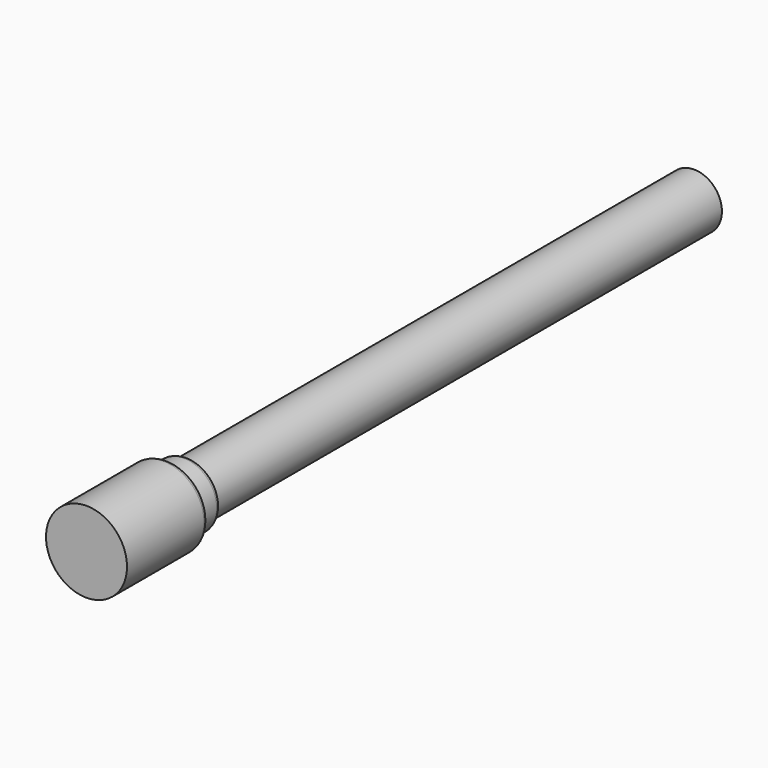
from build123d import *

# Parameters (mm, degrees)
F0_R     = 11
F1_DEPTH = 250
F2_R     = 13
F2_R_2   = 11
F3_DEPTH = 10
F4_R     = 1.99999
F5_R     = 16
F5_R_2   = 13
F6_DEPTH = 40
F7_R     = 2


# Not quite as in the source:
# - a fillet or chamfer is up to 0.001 mm smaller than in the source, because OpenCascade refuses the exact size


with BuildPart() as f1:
    # F0 (on Front) → F1 (new body)
    with BuildSketch(Plane.XZ):
        Circle(F0_R)
    extrude(amount=F1_DEPTH)

    # F2 (on face) → F3 (join)
    with BuildSketch(Plane.XZ.offset(250)):
        Circle(F2_R)
        Circle(F2_R_2, mode=Mode.SUBTRACT)
        Circle(F2_R_2)
    extrude(amount=F3_DEPTH)

    # F4 (radius 2 in the source; OpenCascade refuses exactly that, so slightly less here)
    f4_edges = [f1.edges().sort_by_distance(p)[0] for p in [
        (-13, -250, 0),
    ]]
    fillet(f4_edges, radius=F4_R)

    # F5 (on face) → F6 (join)
    with BuildSketch(Plane.XZ.offset(260)):
        Circle(F5_R)
        Circle(F5_R_2, mode=Mode.SUBTRACT)
        Circle(F5_R_2)
    extrude(amount=F6_DEPTH)

    # F7
    f7_edges = [f1.edges().sort_by_distance(p)[0] for p in [
        (-16, -260, 0),
    ]]
    fillet(f7_edges, radius=F7_R)


solid = f1.part
